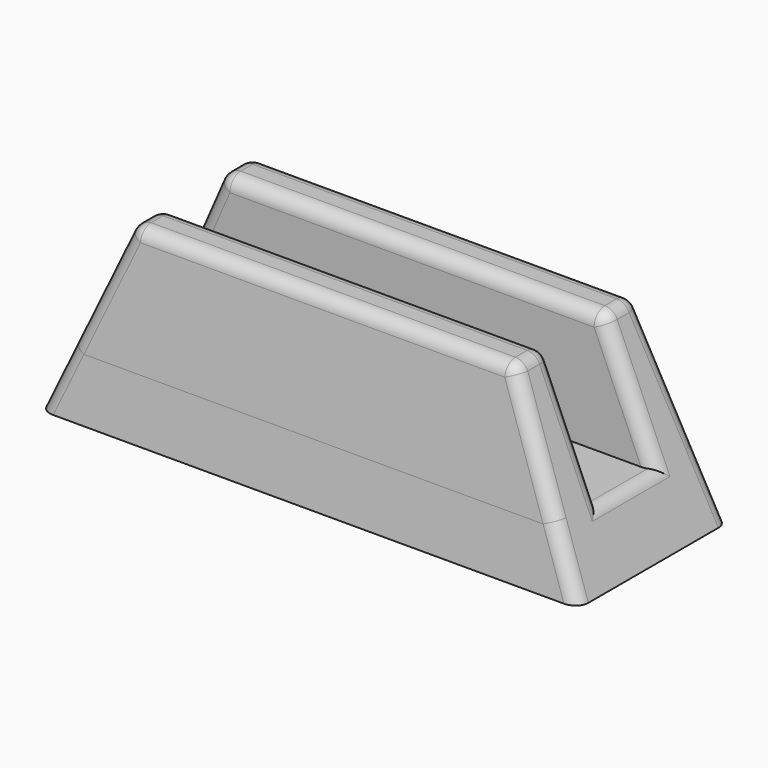
from build123d import *

# Parameters (mm, degrees)
F1_DEPTH = 200
F2_W     = 158.6660303175
F2_H     = 22.1358127892
F3_DEPTH = 20
F5_DEPTH = 75
F7_R     = 5


# Not quite as in the source:
# - a feature of the source that left no trace in its solid (it failed there, or was rolled back) is left out
# - a feature names something its author has since deleted; it is built from what else it names


with BuildPart() as f1:
    # F0 (on Right) → F1 (new body)
    with BuildSketch(Plane.YZ):
        Polygon((12.9773180083, 11), (-13.0226819917, 11), (-32.7089403555, 11), (-35, -11), (35, -11), (32.6940447192, 11), align=None)
        Polygon((12.9773180083, 56), (12.9773180083, 11), (32.6940447192, 11), (27.9773180083, 56), align=None)
        Polygon((-32.7089403555, 11), (-13.0226819917, 11), (-13.0226819917, 56), (-28.0226819917, 56), align=None)
    extrude(amount=F1_DEPTH)

    # F2 (on face) → F3 (cut)
    with BuildSketch(Plane(origin=(0, 0, -11), x_dir=(1, 0, 0), z_dir=(0, 0, -1))):
        with Locations((100, 0)):
            Rectangle(F2_W, F2_H)
    extrude(amount=-F3_DEPTH, mode=Mode.SUBTRACT)

    # F4 (on Front) → F5 (cut, symmetric)
    with BuildSketch(Plane.XZ):
        Polygon((0, -11), (29.1324291224, 56), (0, 56), align=None)
        Polygon((200, -11), (200, 56), (170.8675708776, 56), align=None)
    extrude(amount=F5_DEPTH, both=True, mode=Mode.SUBTRACT)

    # F7
    f7_edges = [f1.edges().sort_by_distance(p)[0] for p in [
        (29.132429, 20.477318, 56),
        (9.565872, -0.022682, 11),
        (190.434128, -0.022682, 11),
        (14.566215, -31.511341, 22.5),
        (29.132429, -20.522682, 56),
        (19.349151, -13.022682, 33.5),
        (19.349151, 12.977318, 33.5),
        (14.566215, 31.488659, 22.5),
        (100, -13.022682, 56),
        (180.650849, -13.022682, 33.5),
        (170.867571, 20.477318, 56),
        (180.650849, 12.977318, 33.5),
        (170.867571, -20.522682, 56),
        (185.433785, -31.511341, 22.5),
        (185.433785, 31.488659, 22.5),
        (100, 12.977318, 56),
        (100, -28.022682, 56),
        (100, 27.977318, 56),
    ]]
    fillet(f7_edges, radius=F7_R)


solid = f1.part
